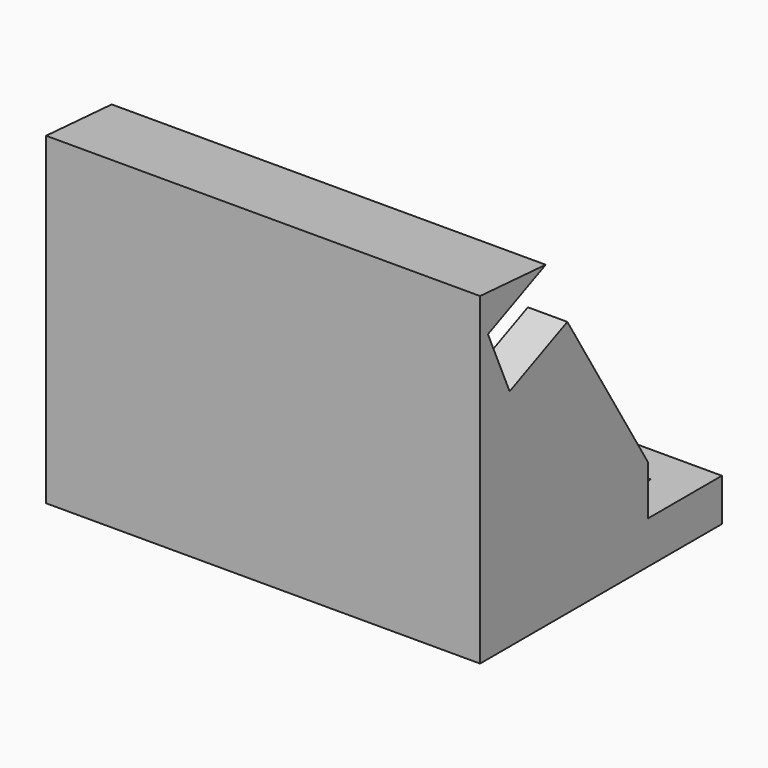
from build123d import *

# Parameters (mm, degrees)
F1_DEPTH = 22
F2_T     = 2
F3_DEPTH = 4
F4_DEPTH = 2.5


# Not quite as in the source:
# - a shell that OpenCascade refuses in one call is made with other operations: the cavity is built on its own and cut out
# - a feature names something its author has since deleted; it is built from what else it names


with BuildPart() as f1:
    # F0 (on Right) → F1 (new body)
    with BuildSketch(Plane.YZ):
        Polygon((-45.7758642733, 0), (-30.4509963948, 0), (-30.4525867105, 4.6551725827), (-35.1306907833, 4.6535744332), (-40.2460545301, 13.0035160109), (-41.6182950139, 16.1101743579), (-45.7758642733, 16.402374953), align=None)
    extrude(amount=F1_DEPTH)

    # F2: shell of thickness 2, made by hand


with BuildPart() as f2_core1:
    # F2_t2: copy of F1
    add(f1.part)

    # the walls: a layer under each face that stays
    f2_faces = [f2_core1.faces().sort_by_distance(p)[0] for p in [
        (11, -40.932174772, 14.5568451844),
        (11, -43.6970796436, 16.2562746555),
        (11, -45.7758642733, 8.2011874765),
        (11, -38.1134303341, 0),
        (11, -30.4517915527, 2.3275862914),
        (11, -32.7916387469, 4.6543735079),
        (0, -38.1134303341, 8.2011874765),
        (22, -38.1134303341, 8.2011874765),
    ]]
    thicken(f2_faces, amount=-F2_T, mode=Mode.SUBTRACT)


with BuildPart() as f1_1:
    add(f1.part)

    # what is left inside the walls is the cavity
    f2_cavity = [f2_core1.part.solids().sort_by_distance(p)[0] for p in [
        (14, -43.755864, 8.128439),
    ]]
    add(f2_cavity, mode=Mode.SUBTRACT)

    # F3 (cut): a face of the model
    f3_faces = [f1_1.faces().sort_by_distance(p)[0] for p in [
        (11, -40.932174772, 14.5568451844),
    ]]
    extrude(f3_faces, amount=-F3_DEPTH, mode=Mode.SUBTRACT)

    # F4 (cut): a face of the model
    f4_faces = [f1_1.faces().sort_by_distance(p)[0] for p in [
        (11, -32.7916387469, 4.6543735079),
    ]]
    extrude(f4_faces, amount=-F4_DEPTH, mode=Mode.SUBTRACT)


solid = f1_1.part
